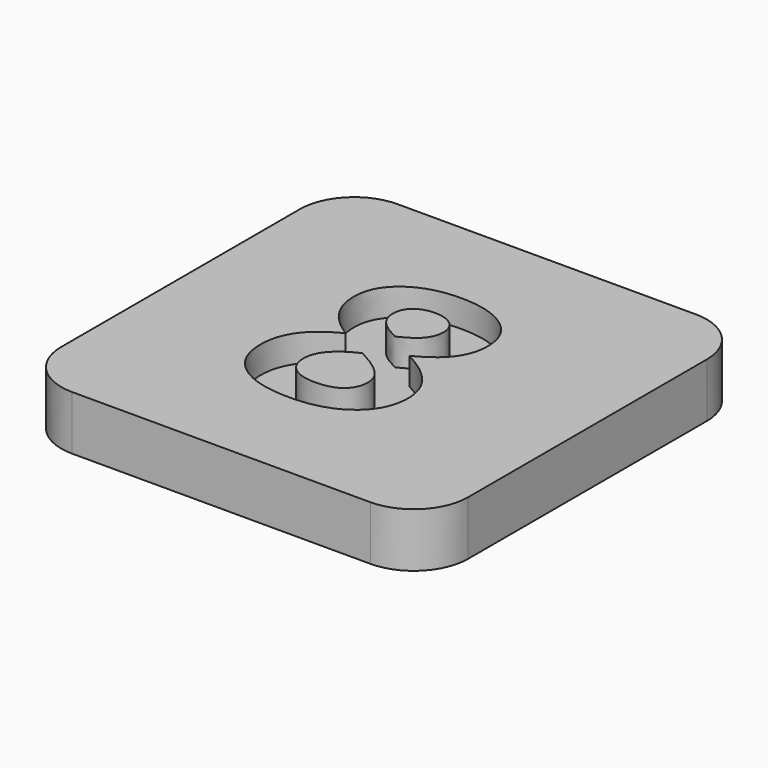
from build123d import *

# Parameters (mm, degrees)
F0_W         = 38.1
F0_H         = 38.1
F1_DEPTH     = 5.08
F2_TEXT_SIZE = 27.4737389496
F3_DEPTH     = 2.54
F4_R         = 5.08


# Not quite as in the source:
# - Text() gives the source's letters only with a copy of the font that has no kerning and outlines rounded to 1/6400 em; it was checked with that copy


with BuildPart() as f1:
    # F0 (on Top) → F1 (new body)
    with BuildSketch(Plane.XY):
        Rectangle(F0_W, F0_H)
    extrude(amount=F1_DEPTH)

    # F2 (on face) → F3 (cut)
    with BuildSketch(Plane.XY.offset(5.08)):
        with Locations((-8.89, -9.525)):
            Text('8', F2_TEXT_SIZE, font='Open Sans', font_style=FontStyle.BOLD, text_align=(TextAlign.LEFT, TextAlign.BOTTOM))
    extrude(amount=-F3_DEPTH, mode=Mode.SUBTRACT)

    # F4
    f4_edges = [f1.edges().sort_by_distance(p)[0] for p in [
        (-19.05, -19.05, 2.54),
        (19.05, -19.05, 2.54),
        (19.05, 19.05, 2.54),
        (-19.05, 19.05, 2.54),
    ]]
    fillet(f4_edges, radius=F4_R)


solid = f1.part
